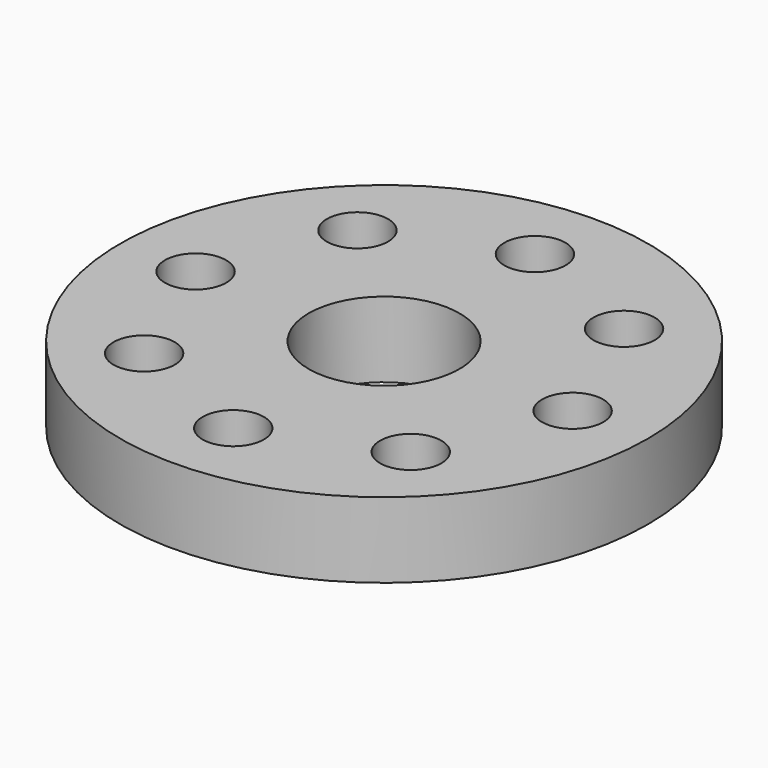
from build123d import *

# Parameters (mm, degrees)
F0_R     = 88.9
F1_DEPTH = 25.4
F2_D     = 20.6375
F4_D     = 50.8


# Not quite as in the source:
# - a feature names something its author has since deleted; it is built from what else it names


with BuildPart() as f1:
    # F0 (on Top) → F1 (new body)
    with BuildSketch(Plane.XY):
        Circle(F0_R)
    extrude(amount=F1_DEPTH)

    # F2 (through all)
    with Locations(Plane(origin=(0, 0, 0), x_dir=(1, 0, 0), z_dir=(0, 0, -1))):
        with Locations((0, -63.5), (-44.9012806053, -44.9012806053), (-63.5, 0), (-44.9012806053, 44.9012806053), (44.9012806053, 44.9012806053), (0, 63.5), (63.5, 0), (44.9012806053, -44.9012806053)):
            Hole(F2_D / 2)

    # F4 (through all)
    with Locations(Plane.XY.offset(25.4)):
        with Locations((0, 0)):
            Hole(F4_D / 2)


solid = f1.part
